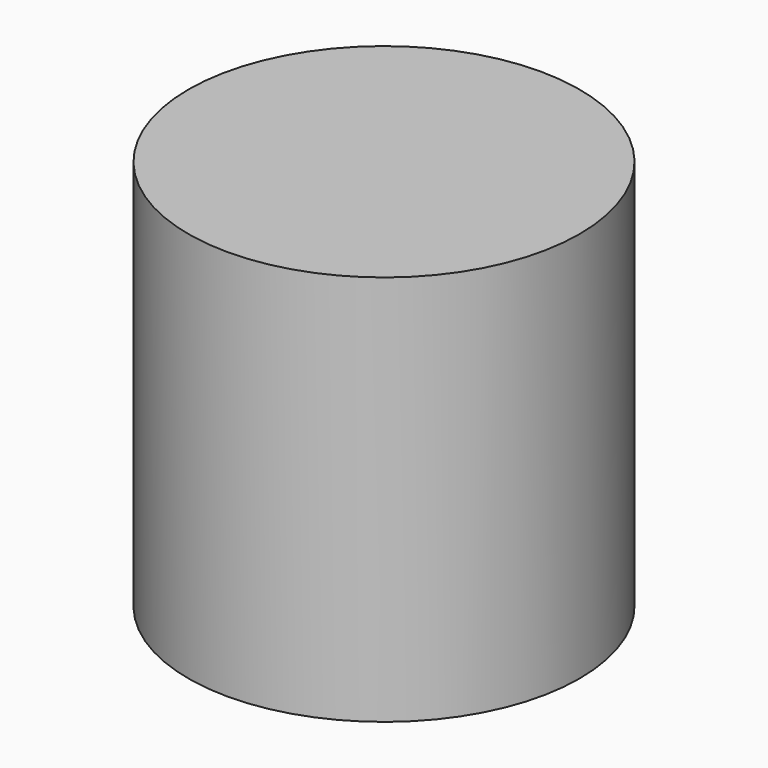
from build123d import *

# Parameters (mm, degrees)
F0_R     = 12.7
F1_DEPTH = 25.4


# Not quite as in the source:
# - the program builds the solid bodies; features that only make, move or delete a surface that nothing else refers to are left out


with BuildPart() as f1:
    # F0 (on Top) → F1 (new body)
    with BuildSketch(Plane.XY):
        Circle(F0_R)
    extrude(amount=F1_DEPTH)


solid = f1.part
